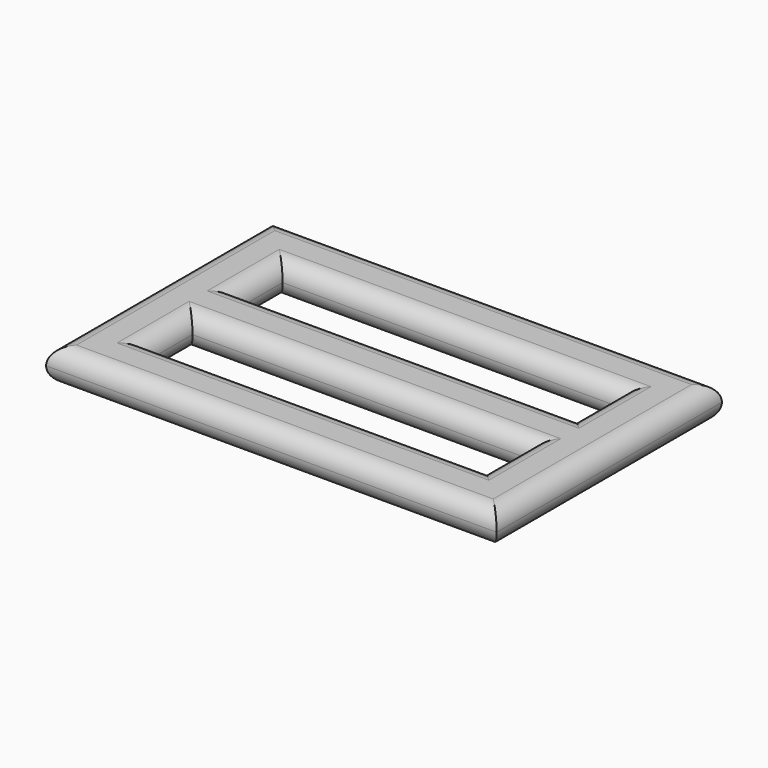
from build123d import *

# Parameters (mm, degrees)
F0_W     = 40
F0_H     = 25
F0_W_2   = 30
F0_H_2   = 5
F1_DEPTH = 3
F2_R     = 1.49999


# Not quite as in the source:
# - a fillet or chamfer is up to 0.001 mm smaller than in the source, because OpenCascade refuses the exact size


with BuildPart() as f1:
    # F0 (on Top) → F1 (new body)
    with BuildSketch(Plane.XY):
        Rectangle(F0_W, F0_H)
        with Locations((0, -5)):
            Rectangle(F0_W_2, F0_H_2, mode=Mode.SUBTRACT)
        with Locations((0, 5)):
            Rectangle(F0_W_2, F0_H_2, mode=Mode.SUBTRACT)
    extrude(amount=F1_DEPTH)

    # F2 (radius 1.5 in the source; OpenCascade refuses exactly that, so slightly less here)
    f2_edges = [f1.edges().sort_by_distance(p)[0] for p in [
        (0, -12.5, 3),
        (-20, 0, 3),
        (0, 12.5, 3),
        (20, 0, 3),
        (0, -12.5, 0),
        (20, 0, 0),
        (-20, 0, 0),
        (0, 12.5, 0),
        (0, 2.5, 3),
        (0, 7.5, 3),
        (15, 5, 3),
        (15, -5, 3),
        (0, -7.5, 3),
        (0, -2.5, 3),
        (-15, -5, 3),
        (-15, 5, 3),
        (0, 2.5, 0),
        (15, 5, 0),
        (0, 7.5, 0),
        (-15, 5, 0),
        (-15, -5, 0),
        (0, -2.5, 0),
        (15, -5, 0),
        (0, -7.5, 0),
    ]]
    fillet(f2_edges, radius=F2_R)


solid = f1.part
